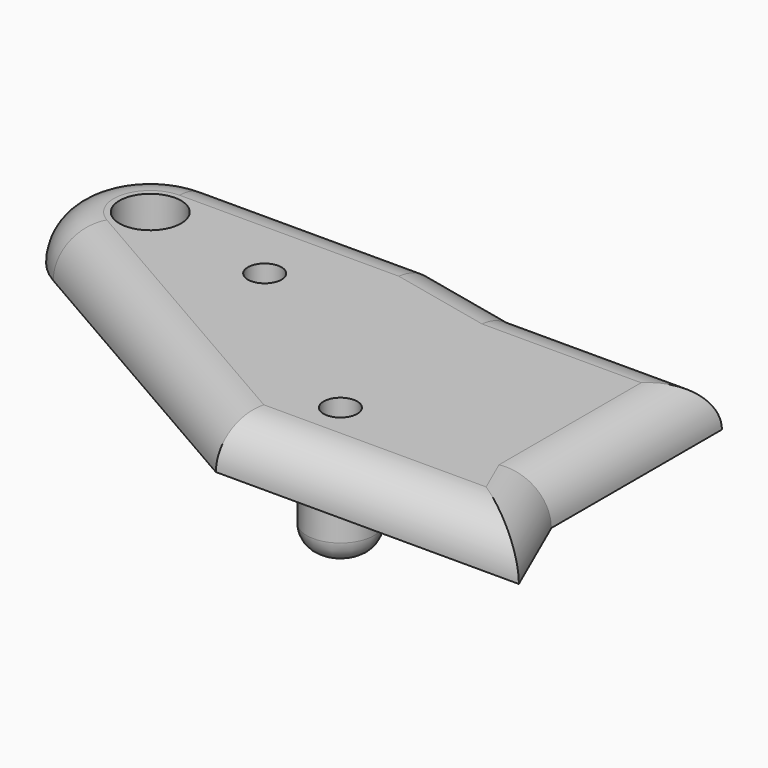
from build123d import *

# Parameters (mm, degrees)
F0_R     = 3
F0_R_2   = 2.75
F0_R_3   = 1.5
F1_DEPTH = 4
F2_DEPTH = 7
F4_R     = 3.99999


# Not quite as in the source:
# - a fillet or chamfer that OpenCascade refuses, or shapes differently, is made with other operations: its cross-section is extruded or revolved along the edge and cut away or added
# - a fillet or chamfer is up to 0.001 mm smaller than in the source, because OpenCascade refuses the exact size


with BuildPart() as f1:
    # F0 (on Top) → F1 (new body)
    with BuildSketch(Plane.XY):
        with BuildLine():
            Line((0, 0), (23.5013441249, 0))
            Line((23.5013441249, 0), (23.5013441249, 8))
            Line((23.5013441249, 8), (23.5013441249, 27))
            Line((23.5013441249, 27), (5.7513441249, 27))
            Line((5.7513441249, 27), (-3.2486558751, 29))
            Line((-3.2486558751, 29), (-23.2486558751, 29))
            ThreePointArc((-23.2486558751, 29), (-30.2527750248, 23.6221150973), (-26.8659020001, 15.4668455))
            Line((-26.8659020001, 15.4668455), (0, 0))
        make_face()
        with Locations((5.5013441249, 7)):
            Circle(F0_R, mode=Mode.SUBTRACT)
        with Locations((-23.2486558751, 21.75)):
            Circle(F0_R_2, mode=Mode.SUBTRACT)
        with Locations((-11.2486558751, 19.5)):
            Circle(F0_R, mode=Mode.SUBTRACT)
        Polygon((23.5013441249, 8), (23.5013441249, 0), (27.0013441249, 0), align=None)
        with Locations((-11.2486558751, 19.5)):
            Circle(F0_R)
        with Locations((-11.2486558751, 19.5)):
            Circle(F0_R_3, mode=Mode.SUBTRACT)
        with Locations((5.5013441249, 7)):
            Circle(F0_R)
        with Locations((5.5013441249, 7)):
            Circle(F0_R_3, mode=Mode.SUBTRACT)
    extrude(amount=F1_DEPTH)

    # F0 (on Top) → F2 (join)
    with BuildSketch(Plane.XY):
        with Locations((-11.2486558751, 19.5)):
            Circle(F0_R)
        with Locations((-11.2486558751, 19.5)):
            Circle(F0_R_3, mode=Mode.SUBTRACT)
        with Locations((5.5013441249, 7)):
            Circle(F0_R)
        with Locations((5.5013441249, 7)):
            Circle(F0_R_3, mode=Mode.SUBTRACT)
    extrude(amount=-F2_DEPTH)

    # F3: fillet of radius 2 on 2 edges, made by hand

    # F3_s1 → F3_t2 (revolve, cut)
    with BuildSketch(Plane.XZ.offset(-19.5)):
        with BuildLine():
            ThreePointArc((-9.7486558751, -7), (-8.667517045, -6.2882531983), (-8.2486558751, -5.0635083269))
            Line((-8.2486558751, -5.0635083269), (-8.2486558751, -7))
            Line((-8.2486558751, -7), (-9.7486558751, -7))
        make_face()
    revolve(axis=Axis((-11.2486558751, 19.5, -7), (0, 0, 1)), mode=Mode.SUBTRACT)

    # F3_s3 → F3_t4 (revolve, cut)
    with BuildSketch(Plane.XZ.offset(-7)):
        with BuildLine():
            ThreePointArc((7.0013441249, -7), (8.082482955, -6.2882531983), (8.5013441249, -5.0635083269))
            Line((8.5013441249, -5.0635083269), (8.5013441249, -7))
            Line((8.5013441249, -7), (7.0013441249, -7))
        make_face()
    revolve(axis=Axis((5.5013441249, 7, -7), (0, 0, 1)), mode=Mode.SUBTRACT)

    # F4 (radius 4 in the source; OpenCascade refuses exactly that, so slightly less here)
    f4_edges = [f1.edges().sort_by_distance(p)[0] for p in [
        (-13.248656, 29, 4),
        (13.500672, 0, 4),
        (25.251344, 4, 4),
        (23.501344, 17.5, 4),
        (1.251344, 28, 4),
        (14.626344, 27, 4),
        (-13.432951, 7.733423, 4),
        (-30.252775, 23.622115, 4),
    ]]
    fillet(f4_edges, radius=F4_R)


solid = f1.part
